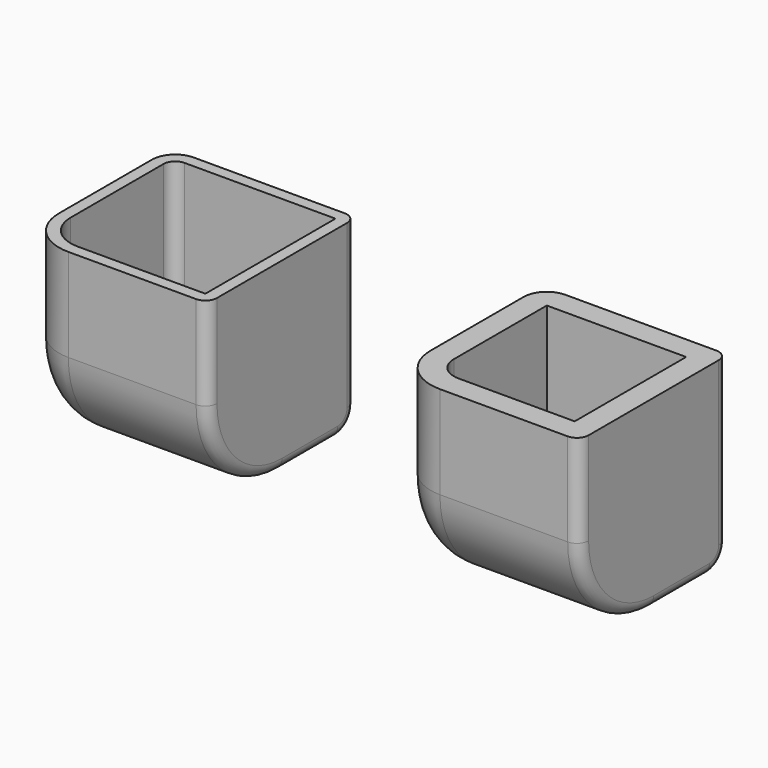
from build123d import *

# Parameters (mm, degrees)
F0_W     = 12.7
F0_H     = 12.7
F1_DEPTH = 12.7
F2_R     = 6.35
F3_R     = 3.175
F4_R     = 1.5875
F5_R     = 0.79375
F7_T     = 0.79375
F8_T     = 1.5875


# Not quite as in the source:
# - a shell that OpenCascade refuses in one call is made with other operations: the cavity is built on its own and cut out


with BuildPart() as f1:
    # F0 (on Top) → F1 (new body)
    with BuildSketch(Plane.XY):
        Rectangle(F0_W, F0_H)
    extrude(amount=F1_DEPTH)

    # F2
    f2_edges = [f1.edges().sort_by_distance(p)[0] for p in [
        (0, -6.35, 0),
    ]]
    fillet(f2_edges, radius=F2_R)

    # F3
    f3_edges = [f1.edges().sort_by_distance(p)[0] for p in [
        (-6.35, 3.175, 0),
    ]]
    fillet(f3_edges, radius=F3_R)

    # F4
    f4_edges = [f1.edges().sort_by_distance(p)[0] for p in [
        (1.5875, 6.35, 0),
    ]]
    fillet(f4_edges, radius=F4_R)

    # F5
    f5_edges = [f1.edges().sort_by_distance(p)[0] for p in [
        (6.35, 2.38125, 0),
    ]]
    fillet(f5_edges, radius=F5_R)


with BuildPart() as f6_1:
    # F6: copy of F1
    add(f1.part.moved(Location((25.4, 0, 0))))

    # F8: shell of thickness 1.5875, made by hand


with BuildPart() as f1_1:
    add(f1.part)

    # F7: shell of thickness 0.79375, made by hand


with BuildPart() as f7_core1:
    # F7_t2: copy of F1
    add(f1_1.part)

    # the walls: a layer under each face that stays
    f7_faces = [f7_core1.faces().sort_by_distance(p)[0] for p in [
        (0.396875, 6.35, 7.14375),
        (-5.8850320151, 5.8850320151, 7.9375),
        (6.35, 0, 6.746875),
        (-6.35, 0.79375, 7.9375),
        (-5.4200640303, -5.4200640303, 9.525),
        (1.190625, -6.35, 9.525),
        (1.190625, 5.8850320151, 0.4649679849),
        (-5.0912820151, 5.8850320151, 1.2587179849),
        (-5.4200640303, 2.38125, 0.9299359697),
        (-5.4200640303, -3.8325640303, 2.5174359697),
        (1.190625, -4.4901280605, 1.8598719395),
        (1.190625, 2.38125, 0),
    ]]
    thicken(f7_faces, amount=-F7_T, mode=Mode.SUBTRACT)


with BuildPart() as f1_2:
    add(f1_1.part)

    # what is left inside the walls is the cavity
    f7_cavity = [f7_core1.part.solids().sort_by_distance(p)[0] for p in [
        (5.548312, 0, 8.73125),
    ]]
    add(f7_cavity, mode=Mode.SUBTRACT)


with BuildPart() as f8_core1:
    # F8_t2: copy of F6_1
    add(f6_1.part)

    # the walls: a layer under each face that stays
    f8_faces = [f8_core1.faces().sort_by_distance(p)[0] for p in [
        (25.796875, 6.35, 7.14375),
        (31.75, 0, 6.746875),
        (19.05, 0.79375, 7.9375),
        (19.9799359697, -5.4200640303, 9.525),
        (26.590625, -6.35, 9.525),
        (19.9799359697, 2.38125, 0.9299359697),
        (19.9799359697, -3.8325640303, 2.5174359697),
        (26.590625, -4.4901280605, 1.8598719395),
        (26.590625, 2.38125, 0),
    ]]
    thicken(f8_faces, amount=-F8_T, mode=Mode.SUBTRACT)


with BuildPart() as f6_1_1:
    add(f6_1.part)

    # what is left inside the walls is the cavity
    f8_cavity = [f8_core1.part.solids().sort_by_distance(p)[0] for p in [
        (25.4, 4.746625, 8.995833),
    ]]
    add(f8_cavity, mode=Mode.SUBTRACT)


solid = Compound([f1_2.part, f6_1_1.part])
